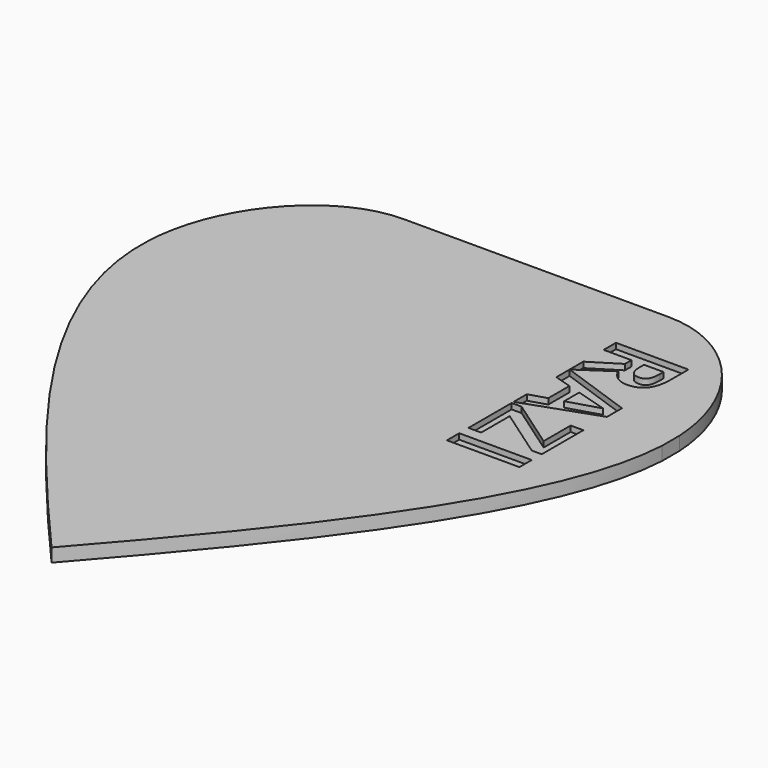
from build123d import *

# Parameters (mm, degrees)
F1_DEPTH     = 0.71
F3_TEXT_SIZE = 5.3683769048
F4_DEPTH     = 0.3


# Not quite as in the source:
# - Text() gives the source's letters only with a copy of the font that has no kerning and outlines rounded to 1/6400 em; it was checked with that copy


with BuildPart() as f1:
    # F0 (on Top) → F1 (new body)
    with BuildSketch(Plane.XY):
        with BuildLine():
            add(Edge.make_bspline(
                [(-14, 6.8524436895), (-13.618903379, -0.0072139084), (-6.62557914, -8.4279095543), (0, -16)],
                knots=[0.4152054373, 0.4152054373, 0.4152054373, 0.4152054373, 1, 1, 1, 1], degree=3))
            add(Edge.make_bspline(
                [(14, 6.8524436895), (13.618903379, -0.0072139084), (6.62557914, -8.4279095543), (0, -16)],
                knots=[0.4152054373, 0.4152054373, 0.4152054373, 0.4152054373, 1, 1, 1, 1], degree=3))
            Line((14, 6.8524436895), (14, 8))
            add(Edge.make_bspline(
                [(7, 16), (10.5, 16), (13.7461012471, 12.3623970458), (14, 8)],
                knots=[0, 0, 0, 0, 0.3821578685, 0.3821578685, 0.3821578685, 0.3821578685], degree=3))
            Line((7, 16), (-7, 16))
            add(Edge.make_bspline(
                [(-7, 16), (-10.5, 16), (-13.7461012471, 12.3623970458), (-14, 8)],
                knots=[0, 0, 0, 0, 0.3821578685, 0.3821578685, 0.3821578685, 0.3821578685], degree=3))
            Line((-14, 8), (-14, 6.8524436895))
        make_face()
    extrude(amount=F1_DEPTH)

    # F3 (on offset) → F4 (cut)
    with BuildSketch(Plane.XY.offset(0.71)):
        with Locations(Location((6.7638242238, 13.323095169), (0, 0, -90))):
            Text('RAZI', F3_TEXT_SIZE, font='Open Sans', font_style=FontStyle.BOLD, text_align=(TextAlign.LEFT, TextAlign.BOTTOM))
    extrude(amount=-F4_DEPTH, mode=Mode.SUBTRACT)


solid = f1.part
